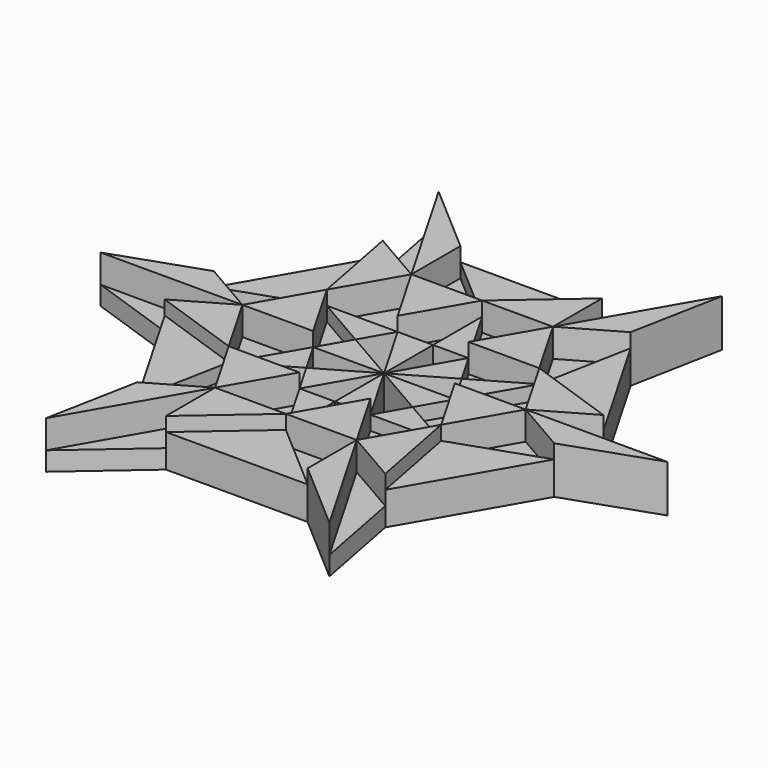
from build123d import *

# Parameters (mm, degrees)
F1_DEPTH = 6.35
F2_DEPTH = 4.445
F3_DEPTH = 2.54


# Not quite as in the source:
# - a feature names something its author has since deleted; it is built from what else it names


with BuildPart() as f1:
    # F0 (on Top) → F1 (new body)
    with BuildSketch(Plane.XY):
        Polygon((-26.19375, 4.1244459855), (-38.1, 0), (-19.05, 0), align=None)
    extrude(amount=F1_DEPTH)


with BuildPart() as f1b:
    # F0 (on Top) → F1, piece 2 (new body)
    with BuildSketch(Plane.XY):
        Polygon((26.19375, -4.1244459855), (38.1, 0), (19.05, 0), align=None)
    extrude(amount=F1_DEPTH)


with BuildPart() as f1c:
    # F0 (on Top) → F1, piece 3 (new body)
    with BuildSketch(Plane.XY):
        Polygon((16.66875, 20.6222299276), (19.05, 32.9955678842), (9.525, 16.4977839421), align=None)
    extrude(amount=F1_DEPTH)


with BuildPart() as f1d:
    # F0 (on Top) → F1, piece 4 (new body)
    with BuildSketch(Plane.XY):
        Polygon((-9.525, 24.7466759131), (-19.05, 32.9955678842), (-9.525, 16.4977839421), align=None)
    extrude(amount=F1_DEPTH)


with BuildPart() as f1e:
    # F0 (on Top) → F1, piece 5 (new body)
    with BuildSketch(Plane.XY):
        Polygon((9.525, -24.7466759131), (19.05, -32.9955678842), (9.525, -16.4977839421), align=None)
    extrude(amount=F1_DEPTH)


with BuildPart() as f1f:
    # F0 (on Top) → F1, piece 6 (new body)
    with BuildSketch(Plane.XY):
        Polygon((-16.66875, -20.6222299276), (-19.05, -32.9955678842), (-9.525, -16.4977839421), align=None)
    extrude(amount=F1_DEPTH)


with BuildPart() as f1g:
    # F0 (on Top) → F1, piece 7 (new body)
    with BuildSketch(Plane.XY):
        Polygon((-14.2875, -8.248891971), (-19.05, 0), (-26.19375, -4.1244459855), align=None)
    extrude(amount=F1_DEPTH)


with BuildPart() as f1h:
    # F0 (on Top) → F1, piece 8 (new body)
    with BuildSketch(Plane.XY):
        Polygon((-14.2875, 8.248891971), (-9.525, 16.4977839421), (-16.66875, 20.6222299276), align=None)
    extrude(amount=F1_DEPTH)


with BuildPart() as f1i:
    # F0 (on Top) → F1, piece 9 (new body)
    with BuildSketch(Plane.XY):
        Polygon((9.525, 24.7466759131), (0, 16.4977839421), (9.525, 16.4977839421), align=None)
    extrude(amount=F1_DEPTH)


with BuildPart() as f1j:
    # F0 (on Top) → F1, piece 10 (new body)
    with BuildSketch(Plane.XY):
        Polygon((14.2875, 8.248891971), (19.05, 0), (26.19375, 4.1244459855), align=None)
    extrude(amount=F1_DEPTH)


with BuildPart() as f1k:
    # F0 (on Top) → F1, piece 11 (new body)
    with BuildSketch(Plane.XY):
        Polygon((16.66875, -20.6222299276), (14.2875, -8.248891971), (9.525, -16.4977839421), align=None)
    extrude(amount=F1_DEPTH)


with BuildPart() as f1l:
    # F0 (on Top) → F1, piece 12 (new body)
    with BuildSketch(Plane.XY):
        Polygon((-9.525, -24.7466759131), (0, -16.4977839421), (-9.525, -16.4977839421), align=None)
    extrude(amount=F1_DEPTH)


with BuildPart() as f1m:
    # F0 (on Top) → F1, piece 13 (new body)
    with BuildSketch(Plane.XY):
        Polygon((-4.7625, -8.248891971), (-14.2875, -8.248891971), (-9.525, -16.4977839421), align=None)
    extrude(amount=F1_DEPTH)


with BuildPart() as f1n:
    # F0 (on Top) → F1, piece 14 (new body)
    with BuildSketch(Plane.XY):
        Polygon((14.2875, 8.248891971), (9.525, 16.4977839421), (4.7625, 8.248891971), align=None)
    extrude(amount=F1_DEPTH)


with BuildPart() as f1o:
    # F0 (on Top) → F1, piece 15 (new body)
    with BuildSketch(Plane.XY):
        Polygon((14.2875, -8.248891971), (19.05, 0), (9.525, 0), align=None)
    extrude(amount=F1_DEPTH)


with BuildPart() as f1p:
    # F0 (on Top) → F1, piece 16 (new body)
    with BuildSketch(Plane.XY):
        Polygon((0, -16.4977839421), (9.525, -16.4977839421), (4.7625, -8.248891971), align=None)
    extrude(amount=F1_DEPTH)


with BuildPart() as f1q:
    # F0 (on Top) → F1, piece 17 (new body)
    with BuildSketch(Plane.XY):
        Polygon((-4.7625, 8.248891971), (0, 16.4977839421), (-9.525, 16.4977839421), align=None)
    extrude(amount=F1_DEPTH)


with BuildPart() as f1r:
    # F0 (on Top) → F1, piece 18 (new body)
    with BuildSketch(Plane.XY):
        Polygon((-14.2875, 8.248891971), (-19.05, 0), (-9.525, 0), align=None)
    extrude(amount=F1_DEPTH)


with BuildPart() as f2:
    # F0 (on Top) → F2 (new body)
    with BuildSketch(Plane.XY):
        Polygon((-14.2875, 8.248891971), (-16.66875, 20.6222299276), (-26.19375, 4.1244459855), align=None)
    extrude(amount=F2_DEPTH)


with BuildPart() as f2b:
    # F0 (on Top) → F2, piece 2 (new body)
    with BuildSketch(Plane.XY):
        Polygon((0, 16.4977839421), (0, 24.7466759131), (-9.525, 24.7466759131), align=None)
        Polygon((9.525, 24.7466759131), (0, 24.7466759131), (0, 16.4977839421), align=None)
    extrude(amount=F2_DEPTH)


with BuildPart() as f2c:
    # F0 (on Top) → F2, piece 3 (new body)
    with BuildSketch(Plane.XY):
        Polygon((14.2875, 8.248891971), (26.19375, 4.1244459855), (16.66875, 20.6222299276), align=None)
    extrude(amount=F2_DEPTH)


with BuildPart() as f2d:
    # F0 (on Top) → F2, piece 4 (new body)
    with BuildSketch(Plane.XY):
        Polygon((0, -24.7466759131), (9.525, -24.7466759131), (0, -16.4977839421), align=None)
        Polygon((-9.525, -24.7466759131), (0, -24.7466759131), (0, -16.4977839421), align=None)
    extrude(amount=F2_DEPTH)


with BuildPart() as f2e:
    # F0 (on Top) → F2, piece 5 (new body)
    with BuildSketch(Plane.XY):
        Polygon((-14.2875, -8.248891971), (-26.19375, -4.1244459855), (-16.66875, -20.6222299276), align=None)
    extrude(amount=F2_DEPTH)


with BuildPart() as f2f:
    # F0 (on Top) → F2, piece 6 (new body)
    with BuildSketch(Plane.XY):
        Polygon((16.66875, -20.6222299276), (26.19375, -4.1244459855), (14.2875, -8.248891971), align=None)
    extrude(amount=F2_DEPTH)


with BuildPart() as f2g:
    # F0 (on Top) → F2, piece 7 (new body)
    with BuildSketch(Plane.XY):
        Polygon((7.14375, -4.1244459855), (9.525, 0), (0, 0), align=None)
    extrude(amount=F2_DEPTH)


with BuildPart() as f2h:
    # F0 (on Top) → F2, piece 8 (new body)
    with BuildSketch(Plane.XY):
        Polygon((7.14375, 4.1244459855), (9.525, 0), (14.2875, 8.248891971), align=None)
    extrude(amount=F2_DEPTH)


with BuildPart() as f2i:
    # F0 (on Top) → F2, piece 9 (new body)
    with BuildSketch(Plane.XY):
        Polygon((7.14375, 4.1244459855), (4.7625, 8.248891971), (0, 0), align=None)
    extrude(amount=F2_DEPTH)


with BuildPart() as f2j:
    # F0 (on Top) → F2, piece 10 (new body)
    with BuildSketch(Plane.XY):
        Polygon((4.7625, 8.248891971), (0, 16.4977839421), (0, 8.248891971), align=None)
    extrude(amount=F2_DEPTH)


with BuildPart() as f2k:
    # F0 (on Top) → F2, piece 11 (new body)
    with BuildSketch(Plane.XY):
        Polygon((0, 0), (0, 8.248891971), (-4.7625, 8.248891971), align=None)
    extrude(amount=F2_DEPTH)


with BuildPart() as f2l:
    # F0 (on Top) → F2, piece 12 (new body)
    with BuildSketch(Plane.XY):
        Polygon((-7.14375, 4.1244459855), (-4.7625, 8.248891971), (-14.2875, 8.248891971), align=None)
    extrude(amount=F2_DEPTH)


with BuildPart() as f2m:
    # F0 (on Top) → F2, piece 13 (new body)
    with BuildSketch(Plane.XY):
        Polygon((-9.525, 0), (0, 0), (-7.14375, 4.1244459855), align=None)
    extrude(amount=F2_DEPTH)


with BuildPart() as f2n:
    # F0 (on Top) → F2, piece 14 (new body)
    with BuildSketch(Plane.XY):
        Polygon((-7.14375, -4.1244459855), (-9.525, 0), (-14.2875, -8.248891971), align=None)
    extrude(amount=F2_DEPTH)


with BuildPart() as f2o:
    # F0 (on Top) → F2, piece 15 (new body)
    with BuildSketch(Plane.XY):
        Polygon((-4.7625, -8.248891971), (0, 0), (-7.14375, -4.1244459855), align=None)
    extrude(amount=F2_DEPTH)


with BuildPart() as f2p:
    # F0 (on Top) → F2, piece 16 (new body)
    with BuildSketch(Plane.XY):
        Polygon((-4.7625, -8.248891971), (0, -16.4977839421), (0, -8.248891971), align=None)
    extrude(amount=F2_DEPTH)


with BuildPart() as f2q:
    # F0 (on Top) → F2, piece 17 (new body)
    with BuildSketch(Plane.XY):
        Polygon((4.7625, -8.248891971), (0, 0), (0, -8.248891971), align=None)
    extrude(amount=F2_DEPTH)


with BuildPart() as f2r:
    # F0 (on Top) → F2, piece 18 (new body)
    with BuildSketch(Plane.XY):
        Polygon((4.7625, -8.248891971), (14.2875, -8.248891971), (7.14375, -4.1244459855), align=None)
    extrude(amount=F2_DEPTH)


with BuildPart() as f3:
    # F0 (on Top) → F3 (new body)
    with BuildSketch(Plane.XY):
        Polygon((-19.05, 0), (-38.1, 0), (-26.19375, -4.1244459855), align=None)
    extrude(amount=F3_DEPTH)


with BuildPart() as f3b:
    # F0 (on Top) → F3, piece 2 (new body)
    with BuildSketch(Plane.XY):
        Polygon((-9.525, 16.4977839421), (-19.05, 32.9955678842), (-16.66875, 20.6222299276), align=None)
    extrude(amount=F3_DEPTH)


with BuildPart() as f3c:
    # F0 (on Top) → F3, piece 3 (new body)
    with BuildSketch(Plane.XY):
        Polygon((9.525, 16.4977839421), (19.05, 32.9955678842), (9.525, 24.7466759131), align=None)
    extrude(amount=F3_DEPTH)


with BuildPart() as f3d:
    # F0 (on Top) → F3, piece 4 (new body)
    with BuildSketch(Plane.XY):
        Polygon((19.05, 0), (38.1, 0), (26.19375, 4.1244459855), align=None)
    extrude(amount=F3_DEPTH)


with BuildPart() as f3e:
    # F0 (on Top) → F3, piece 5 (new body)
    with BuildSketch(Plane.XY):
        Polygon((9.525, -16.4977839421), (19.05, -32.9955678842), (16.66875, -20.6222299276), align=None)
    extrude(amount=F3_DEPTH)


with BuildPart() as f3f:
    # F0 (on Top) → F3, piece 6 (new body)
    with BuildSketch(Plane.XY):
        Polygon((-9.525, -16.4977839421), (-19.05, -32.9955678842), (-9.525, -24.7466759131), align=None)
    extrude(amount=F3_DEPTH)


with BuildPart() as f3g:
    # F0 (on Top) → F3, piece 7 (new body)
    with BuildSketch(Plane.XY):
        Polygon((-9.525, -16.4977839421), (-14.2875, -8.248891971), (-16.66875, -20.6222299276), align=None)
    extrude(amount=F3_DEPTH)


with BuildPart() as f3h:
    # F0 (on Top) → F3, piece 8 (new body)
    with BuildSketch(Plane.XY):
        Polygon((-26.19375, 4.1244459855), (-19.05, 0), (-14.2875, 8.248891971), align=None)
    extrude(amount=F3_DEPTH)


with BuildPart() as f3i:
    # F0 (on Top) → F3, piece 9 (new body)
    with BuildSketch(Plane.XY):
        Polygon((-9.525, 16.4977839421), (0, 16.4977839421), (-9.525, 24.7466759131), align=None)
    extrude(amount=F3_DEPTH)


with BuildPart() as f3j:
    # F0 (on Top) → F3, piece 10 (new body)
    with BuildSketch(Plane.XY):
        Polygon((16.66875, 20.6222299276), (9.525, 16.4977839421), (14.2875, 8.248891971), align=None)
    extrude(amount=F3_DEPTH)


with BuildPart() as f3k:
    # F0 (on Top) → F3, piece 11 (new body)
    with BuildSketch(Plane.XY):
        Polygon((26.19375, -4.1244459855), (19.05, 0), (14.2875, -8.248891971), align=None)
    extrude(amount=F3_DEPTH)


with BuildPart() as f3l:
    # F0 (on Top) → F3, piece 12 (new body)
    with BuildSketch(Plane.XY):
        Polygon((9.525, -24.7466759131), (9.525, -16.4977839421), (0, -16.4977839421), align=None)
    extrude(amount=F3_DEPTH)


with BuildPart() as f3m:
    # F0 (on Top) → F3, piece 13 (new body)
    with BuildSketch(Plane.XY):
        Polygon((-9.525, -16.4977839421), (0, -16.4977839421), (-4.7625, -8.248891971), align=None)
    extrude(amount=F3_DEPTH)


with BuildPart() as f3n:
    # F0 (on Top) → F3, piece 14 (new body)
    with BuildSketch(Plane.XY):
        Polygon((-9.525, 0), (-19.05, 0), (-14.2875, -8.248891971), align=None)
    extrude(amount=F3_DEPTH)


with BuildPart() as f3o:
    # F0 (on Top) → F3, piece 15 (new body)
    with BuildSketch(Plane.XY):
        Polygon((-4.7625, 8.248891971), (-9.525, 16.4977839421), (-14.2875, 8.248891971), align=None)
    extrude(amount=F3_DEPTH)


with BuildPart() as f3p:
    # F0 (on Top) → F3, piece 16 (new body)
    with BuildSketch(Plane.XY):
        Polygon((9.525, 16.4977839421), (0, 16.4977839421), (4.7625, 8.248891971), align=None)
    extrude(amount=F3_DEPTH)


with BuildPart() as f3q:
    # F0 (on Top) → F3, piece 17 (new body)
    with BuildSketch(Plane.XY):
        Polygon((9.525, 0), (19.05, 0), (14.2875, 8.248891971), align=None)
    extrude(amount=F3_DEPTH)


with BuildPart() as f3r:
    # F0 (on Top) → F3, piece 18 (new body)
    with BuildSketch(Plane.XY):
        Polygon((9.525, -16.4977839421), (14.2875, -8.248891971), (4.7625, -8.248891971), align=None)
    extrude(amount=F3_DEPTH)


with BuildPart() as f3s:
    # F0 (on Top) → F3, piece 19 (new body)
    with BuildSketch(Plane.XY):
        Polygon((14.2875, -8.248891971), (9.525, 0), (7.14375, -4.1244459855), align=None)
    extrude(amount=F3_DEPTH)


with BuildPart() as f3t:
    # F0 (on Top) → F3, piece 20 (new body)
    with BuildSketch(Plane.XY):
        Polygon((7.14375, 4.1244459855), (14.2875, 8.248891971), (4.7625, 8.248891971), align=None)
    extrude(amount=F3_DEPTH)


with BuildPart() as f3u:
    # F0 (on Top) → F3, piece 21 (new body)
    with BuildSketch(Plane.XY):
        Polygon((0, 8.248891971), (0, 16.4977839421), (-4.7625, 8.248891971), align=None)
    extrude(amount=F3_DEPTH)


with BuildPart() as f3v:
    # F0 (on Top) → F3, piece 22 (new body)
    with BuildSketch(Plane.XY):
        Polygon((-7.14375, 4.1244459855), (-14.2875, 8.248891971), (-9.525, 0), align=None)
    extrude(amount=F3_DEPTH)


with BuildPart() as f3w:
    # F0 (on Top) → F3, piece 23 (new body)
    with BuildSketch(Plane.XY):
        Polygon((-7.14375, -4.1244459855), (-14.2875, -8.248891971), (-4.7625, -8.248891971), align=None)
    extrude(amount=F3_DEPTH)


with BuildPart() as f3x:
    # F0 (on Top) → F3, piece 24 (new body)
    with BuildSketch(Plane.XY):
        Polygon((0, -16.4977839421), (4.7625, -8.248891971), (0, -8.248891971), align=None)
    extrude(amount=F3_DEPTH)


solid = Compound([f1.part, f1b.part, f1c.part, f1d.part, f1e.part, f1f.part, f1g.part, f1h.part, f1i.part, f1j.part, f1k.part, f1l.part, f1m.part, f1n.part, f1o.part, f1p.part, f1q.part, f1r.part, f2.part, f2b.part, f2c.part, f2d.part, f2e.part, f2f.part, f2g.part, f2h.part, f2i.part, f2j.part, f2k.part, f2l.part, f2m.part, f2n.part, f2o.part, f2p.part, f2q.part, f2r.part, f3.part, f3b.part, f3c.part, f3d.part, f3e.part, f3f.part, f3g.part, f3h.part, f3i.part, f3j.part, f3k.part, f3l.part, f3m.part, f3n.part, f3o.part, f3p.part, f3q.part, f3r.part, f3s.part, f3t.part, f3u.part, f3v.part, f3w.part, f3x.part])
